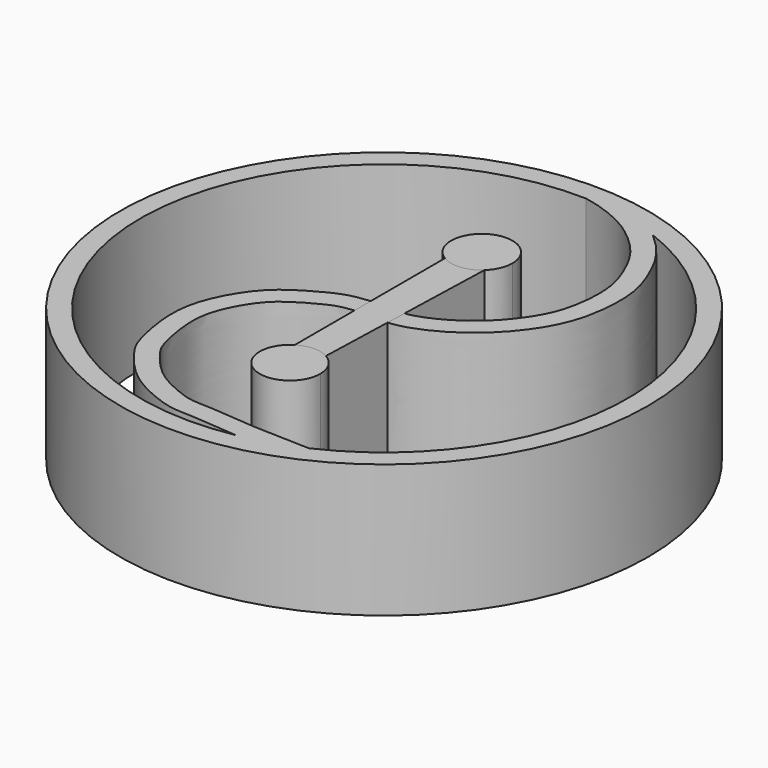
from build123d import *

# Parameters (mm, degrees)
F0_R     = 49.5847500937
F1_DEPTH = 25
F2_DEPTH = 25
F3_DEPTH = 25


# Not quite as in the source:
# - ends of sketch curves that miss each other by under 0.0002 mm in the source are joined
# - the dataset's text gives a spline's control points without its knots; the knots are read off the source's solid


with BuildPart() as f1:
    # F0 (on Top) → F1 (new body)
    with BuildSketch(Plane.XY):
        Circle(F0_R)
        with BuildLine():
            ThreePointArc((8.2176634504, -45.0412423256), (-45.6544875488, -3.451270704), (1.3531451114, 45.7647517323))
            add(Edge.make_bspline(
                [(1.3531451114, 45.7647517323), (3.4585917741, 45.4072790873), (7.3287739419, 44.0760975566), (11.6846514785, 41.8714803536), (17.2036766267, 37.0102398582), (19.8127043525, 31.889785288), (21.8756398334, 26.5737392046), (21.6816430924, 19.8132738016), (20.3466547431, 14.27630368), (17.1645617239, 9.3955679535), (13.7143876632, 5.7022727088), (9.2995178681, 2.6106423405), (5.3224811985, 0.9250643675), (3.6571614218, 0.6611514177), (3.3374725899, 0.6271477481)],
                knots=[0, 0, 0, 0, 0.0402853124, 0.0764233093, 0.1198404643, 0.1588388833, 0.1972733831, 0.2391274731, 0.2779762224, 0.316692206, 0.3531523115, 0.3911291162, 0.4279852066, 0.4371528151, 0.4371528151, 0.4371528151, 0.4371528151], degree=3))
            Line((3.3374725899, 0.6271477481), (3.2173385291, -3.1964079792))
            add(Edge.make_bspline(
                [(16.2617436608, 42.799524033), (16.2630739599, 42.7983750489), (16.6394904754, 42.4732106597), (17.3858142501, 41.7990598434), (18.4668991951, 40.7220167717), (19.3182477466, 39.7747828486), (19.9617151083, 38.9817963008), (20.5615839282, 38.1849818374), (21.2321159557, 37.1896473658), (21.9256201889, 36.0080693011), (22.5259973397, 34.8525285732), (22.9670449801, 33.9153363369), (23.2921740837, 33.1906991104), (23.6162146728, 32.4472971946), (24.0143162389, 31.4754225057), (24.4609945217, 30.2335663035), (24.8545309775, 28.9083557538), (25.1186753026, 27.7330012889), (25.2798865775, 26.7470627199), (25.4025078808, 25.7623445898), (25.4919314322, 24.5315424236), (25.5196391676, 22.5777387036), (25.3996756527, 20.6638298862), (25.1756871665, 18.8523584922), (24.9517875546, 17.5113201902), (24.6589823135, 16.1822687794), (24.2868913691, 14.8644876192), (23.8274995758, 13.5611922588), (23.2686241638, 12.2690224458), (22.636234168, 11.0381846903), (21.7193953434, 9.4746754172), (20.7186347445, 8.0267968339), (19.6941212898, 6.7074239992), (18.6320508644, 5.4397638391), (17.2173630119, 3.9503603048), (15.3457425226, 2.3013523369), (13.2807742381, 0.7790477359), (11.410410694, -0.3634671801), (9.8292090796, -1.1911232786), (8.6167642486, -1.7574183512), (7.5946383314, -2.1736542592), (6.7725118163, -2.466207369), (6.1525609715, -2.6633692461), (5.5289556877, -2.8357079446), (4.8920257832, -2.9805203679), (4.2757329412, -3.0879036918), (3.7163451386, -3.1576990689), (3.3706493697, -3.1862748398), (3.2173385291, -3.1964079792)],
                knots=[0.0937222925, 0.0937222925, 0.0937222925, 0.0937222925, 0.09375, 0.1015625, 0.109375, 0.1171875, 0.12109375, 0.125, 0.1328125, 0.140625, 0.1484375, 0.15625, 0.16015625, 0.1640625, 0.171875, 0.1796875, 0.1875, 0.1953125, 0.19921875, 0.203125, 0.2109375, 0.21875, 0.234375, 0.2421875, 0.25, 0.2578125, 0.265625, 0.2734375, 0.28125, 0.2890625, 0.296875, 0.3125, 0.3203125, 0.328125, 0.34375, 0.359375, 0.375, 0.390625, 0.3984375, 0.40625, 0.4140625, 0.41796875, 0.421875, 0.42578125, 0.4296875, 0.43359375, 0.4375, 0.4407482936, 0.4407482936, 0.4407482936, 0.4407482936], degree=3))
            ThreePointArc((16.2617436608, 42.799524033), (45.7580748478, 1.562718476), (19.1438057271, -41.5903619256))
            add(Edge.make_bspline(
                [(8.5962909195, -41.260151535), (12.1204923737, -41.363963585), (15.6196042728, -41.4865498756), (19.1438057271, -41.5903619256)],
                knots=[0, 0, 0, 0, 10.5526824798, 10.5526824798, 10.5526824798, 10.5526824798], degree=3))
            add(Edge.make_bspline(
                [(-2.9778135602, -3.2238034948), (-3.0993303434, -3.2346970109), (-3.5226099021, -3.2765098979), (-4.0943616278, -3.3525652097), (-4.6705152555, -3.4541250007), (-5.0847144346, -3.5406614246), (-5.4738562213, -3.6363249493), (-5.9558372613, -3.7753006958), (-6.5569469588, -3.9870752932), (-7.2973844437, -4.3047776604), (-7.9556555023, -4.6280032377), (-8.5161141524, -4.9214653693), (-8.9557811473, -5.1586784651), (-9.4151958546, -5.4109743655), (-10.0219149467, -5.7502319027), (-10.7737966428, -6.1856132196), (-11.6435407711, -6.7225847478), (-12.4625455113, -7.2716014199), (-13.2068980448, -7.8239565682), (-13.8680607713, -8.3790853884), (-14.4836619801, -8.9673086499), (-15.0708287585, -9.6073944046), (-15.6482154954, -10.3231261961), (-16.2310819184, -11.1396443892), (-16.8226660281, -12.067261276), (-17.3931826033, -13.069530031), (-17.9227093669, -14.1204821222), (-18.3913882315, -15.1911115172), (-18.7164274723, -16.0743456961), (-18.9297942343, -16.7598333424), (-19.1092008222, -17.4224508448), (-19.3478650369, -18.567657804), (-19.5012310474, -20.2206869085), (-19.4387898602, -22.0343384025), (-19.2699656101, -23.6431361243), (-19.0923777518, -24.8846250566), (-18.8737440335, -26.1095288943), (-18.625273925, -27.270620982), (-18.3605406415, -28.3168815895), (-18.0961057427, -29.1935677611), (-17.8646757486, -29.8180269836), (-17.6428484123, -30.2970196235), (-17.4121763438, -30.7048654836), (-17.1614245266, -31.0964767945), (-16.9309413758, -31.4351019183), (-16.6635644382, -31.8102169288), (-16.2681781339, -32.3424050242), (-15.7106938903, -33.0521363879), (-14.975065644, -33.9229060282), (-14.2063314903, -34.7654131508), (-13.4425929357, -35.5306986434), (-12.7262486355, -36.1712848535), (-12.0138047109, -36.7340261464), (-11.2793708954, -37.2446124357), (-10.4901303857, -37.7297538058), (-9.6147303473, -38.2109085157), (-8.6369747009, -38.7013911181), (-7.6229933124, -39.1651555732), (-6.6109485553, -39.5814499067), (-5.6509540017, -39.9268354746), (-4.7939114132, -40.1807551658), (-4.129478245, -40.3228988125), (-3.4811896898, -40.4095071611), (-2.7268043347, -40.4629905381), (-1.938953452, -40.4930779164), (-1.1935823718, -40.5209796742), (-0.3766220477, -40.5570865106), (0.7204845182, -40.6162695454), (2.1546311267, -40.7083776943), (3.6813461565, -40.8200495776), (5.8114367714, -40.9930475683), (7.4814477769, -41.1477758014), (8.5962909195, -41.260151535)],
                knots=[0.4968401346, 0.4968401346, 0.4968401346, 0.4968401346, 0.5, 0.5078125, 0.51171875, 0.515625, 0.51953125, 0.5234375, 0.53125, 0.5390625, 0.546875, 0.55078125, 0.5546875, 0.55859375, 0.5625, 0.5703125, 0.578125, 0.5859375, 0.59375, 0.6015625, 0.609375, 0.6171875, 0.625, 0.6328125, 0.640625, 0.6484375, 0.65625, 0.6640625, 0.671875, 0.67578125, 0.6796875, 0.6875, 0.703125, 0.71875, 0.7265625, 0.734375, 0.7421875, 0.75, 0.7578125, 0.765625, 0.7734375, 0.78125, 0.7890625, 0.79296875, 0.796875, 0.80078125, 0.8046875, 0.8125, 0.8203125, 0.828125, 0.8359375, 0.84375, 0.8515625, 0.859375, 0.8671875, 0.875, 0.8828125, 0.890625, 0.8984375, 0.90625, 0.9140625, 0.921875, 0.9296875, 0.9375, 0.9453125, 0.94921875, 0.953125, 0.9609375, 0.96875, 0.9765625, 0.984375, 0.9999882092, 0.9999882092, 0.9999882092, 0.9999882092], degree=3))
            Line((-2.9778135602, -3.2238034948), (-2.9778135602, 0.5890359777))
            add(Edge.make_bspline(
                [(-2.9778135602, 0.5890359777), (-4.1586395197, 0.4998871799), (-7.1372789822, 0.0721815891), (-10.9327858042, -1.8493664697), (-15.8365992647, -4.7241770818), (-19.6150340779, -8.8239411152), (-23.2426783003, -16.0189399303), (-23.4442169592, -23.0198313597), (-21.9307663935, -30.3724139092), (-20.290749593, -33.533767655), (-15.9904342503, -38.7653797506), (-11.4707989198, -41.7321009373), (-5.4131902795, -44.2598907097), (-1.1384676764, -44.2508911848), (4.71151601, -44.6877810107), (8.2176634504, -45.0412423256)],
                knots=[0.4943508245, 0.4943508245, 0.4943508245, 0.4943508245, 0.5204850635, 0.5559023161, 0.5940839436, 0.6325130511, 0.6778144538, 0.7214796109, 0.7649859717, 0.7959800891, 0.8371789433, 0.8760457564, 0.9164461256, 0.9499850996, 1, 1, 1, 1], degree=3))
        make_face(mode=Mode.SUBTRACT)
    extrude(amount=F1_DEPTH)


with BuildPart() as f2:
    # F0 (on Top) → F2 (new body)
    with BuildSketch(Plane.XY):
        with BuildLine():
            ThreePointArc((-2.9778135602, 18.0099472335), (0.579881213, 17.2103989752), (3.905499446, 18.705970065))
            ThreePointArc((3.905499446, 18.705970065), (5.2789490027, 20.6308047759), (5.7639747523, 22.9451302439))
            ThreePointArc((5.7639747523, 22.9451302439), (-2.8336692438, 27.9644652159), (-2.9778135602, 18.0099472335))
        make_face()
    extrude(amount=F2_DEPTH)


with BuildPart() as f2b:
    # F0 (on Top) → F2, piece 2 (new body)
    with BuildSketch(Plane.XY):
        with BuildLine():
            ThreePointArc((5.6849669477, -22.0894254744), (4.9051228964, -19.2156442427), (2.7795433476, -17.1302936981))
            ThreePointArc((2.7795433476, -17.1302936981), (-0.1149715971, -16.4056212266), (-2.9778135602, -17.2467531133))
            ThreePointArc((-2.9778135602, -17.2467531133), (-2.7739932886, -27.051663924), (5.6849669477, -22.0894254744))
        make_face()
    extrude(amount=F2_DEPTH)


with BuildPart() as f3:
    # F0 (on Top) → F3 (new body)
    with BuildSketch(Plane.XY):
        with BuildLine():
            add(Edge.make_bspline(
                [(3.3374725899, 0.6271477481), (2.7022433704, 0.5595816578), (1.179826551, 0.5744434161), (-0.8120762037, 0.7033344618), (-2.5254644471, 0.6231869712), (-2.9778135602, 0.5890359777)],
                knots=[0.4371528151, 0.4371528151, 0.4371528151, 0.4371528151, 0.4553690688, 0.4843393577, 0.4943508245, 0.4943508245, 0.4943508245, 0.4943508245], degree=3))
            Line((3.3374725899, 0.6271477481), (3.905499446, 18.705970065))
            ThreePointArc((3.905499446, 18.705970065), (0.579881213, 17.2103989752), (-2.9778135602, 18.0099472335))
            Line((-2.9778135602, 18.0099472335), (-2.9778135602, 0.5890359777))
        make_face()
        with BuildLine():
            Line((2.7795433476, -17.1302936981), (3.2173385291, -3.1964079792))
            add(Edge.make_bspline(
                [(3.2173385291, -3.1964079792), (3.0019201003, -3.2106461438), (2.4372674095, -3.2340467099), (1.7724022915, -3.2260045079), (1.2057258422, -3.207691837), (0.6565254191, -3.1863181965), (-0.002185073, -3.1588329743), (-0.7797750652, -3.1381263752), (-1.5744376242, -3.1401181706), (-2.3217399341, -3.1714582791), (-2.7988903766, -3.2077637137), (-2.9778135602, -3.2238034948)],
                knots=[0.4407482936, 0.4407482936, 0.4407482936, 0.4407482936, 0.4453125, 0.453125, 0.45703125, 0.4609375, 0.46875, 0.4765625, 0.484375, 0.4921875, 0.4968401346, 0.4968401346, 0.4968401346, 0.4968401346], degree=3))
            Line((-2.9778135602, -3.2238034948), (-2.9778135602, -17.2467531133))
            ThreePointArc((-2.9778135602, -17.2467531133), (-0.1149715971, -16.4056212266), (2.7795433476, -17.1302936981))
        make_face()
        with BuildLine():
            Line((3.2173385291, -3.1964079792), (3.3374725899, 0.6271477481))
            add(Edge.make_bspline(
                [(3.3374725899, 0.6271477481), (2.7022433704, 0.5595816578), (1.179826551, 0.5744434161), (-0.8120762037, 0.7033344618), (-2.5254644471, 0.6231869712), (-2.9778135602, 0.5890359777)],
                knots=[0.4371528151, 0.4371528151, 0.4371528151, 0.4371528151, 0.4553690688, 0.4843393577, 0.4943508245, 0.4943508245, 0.4943508245, 0.4943508245], degree=3))
            Line((-2.9778135602, 0.5890359777), (-2.9778135602, -3.2238034948))
            add(Edge.make_bspline(
                [(3.2173385291, -3.1964079792), (3.0019201003, -3.2106461438), (2.4372674095, -3.2340467099), (1.7724022915, -3.2260045079), (1.2057258422, -3.207691837), (0.6565254191, -3.1863181965), (-0.002185073, -3.1588329743), (-0.7797750652, -3.1381263752), (-1.5744376242, -3.1401181706), (-2.3217399341, -3.1714582791), (-2.7988903766, -3.2077637137), (-2.9778135602, -3.2238034948)],
                knots=[0.4407482936, 0.4407482936, 0.4407482936, 0.4407482936, 0.4453125, 0.453125, 0.45703125, 0.4609375, 0.46875, 0.4765625, 0.484375, 0.4921875, 0.4968401346, 0.4968401346, 0.4968401346, 0.4968401346], degree=3))
        make_face()
    extrude(amount=F3_DEPTH)


solid = Compound([f1.part, f2.part, f2b.part, f3.part])
